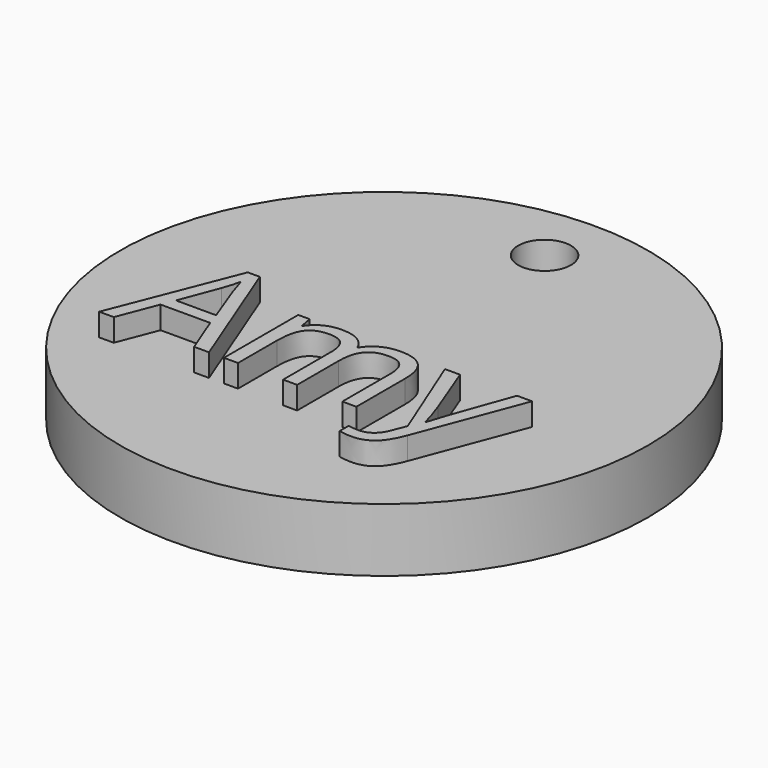
from build123d import *

# Parameters (mm, degrees)
F0_R         = 25
F0_R_2       = 2.5
F1_DEPTH     = 6
F2_TEXT_SIZE = 16.4398664816
F3_DEPTH     = 2.1400707774


# Not quite as in the source:
# - Text() gives the source's letters only with a copy of the font that has no kerning and outlines rounded to 1/6400 em; it was checked with that copy


with BuildPart() as f1:
    # F0 (on Top) → F1 (new body)
    with BuildSketch(Plane.XY):
        Circle(F0_R)
        with Locations((0, 19)):
            Circle(F0_R_2, mode=Mode.SUBTRACT)
    extrude(amount=F1_DEPTH)

    # F2 (on face) → F3 (join)
    with BuildSketch(Plane.XY.offset(6)):
        with Locations((-17.5148796257, -11.8367038667)):
            Text('Amy', F2_TEXT_SIZE, font='Open Sans', text_align=(TextAlign.LEFT, TextAlign.BOTTOM))
    extrude(amount=F3_DEPTH)


solid = f1.part
